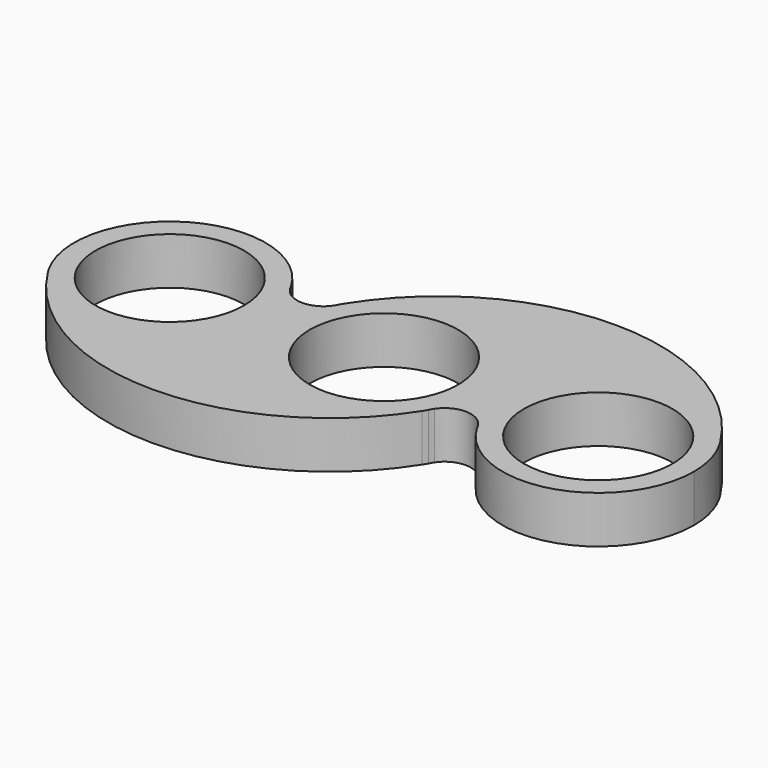
from build123d import *

# Parameters (mm, degrees)
F0_R     = 11.0109
F1_DEPTH = 7


with BuildPart() as f1:
    # F0 (on Top) → F1 (new body)
    with BuildSketch(Plane.XY):
        with BuildLine():
            Line((14.1859, 0), (11.0109, 0))
            ThreePointArc((11.0109, 0), (0, -11.0109), (-11.0109, 0))
            Line((-11.0109, 0), (-14.1859, 0))
            ThreePointArc((-14.1859, 0), (-4.0564627793, -13.5935598182), (11.8660062633, -7.7741658182))
            ThreePointArc((11.8660062633, -7.7741658182), (12.0777532722, -7.4348353952), (12.2853497755, -7.09295))
            ThreePointArc((12.2853497755, -7.09295), (12.4445825488, -6.7642227487), (12.6338376613, -6.4518140673))
            ThreePointArc((12.6338376613, -6.4518140673), (13.7924275689, -3.3179361907), (14.1859, 0))
        make_face()
        with BuildLine():
            ThreePointArc((-11.0109, 0), (0, 11.0109), (11.0109, 0))
            Line((11.0109, 0), (14.1859, 0))
            ThreePointArc((14.1859, 0), (4.0422659472, 13.5977882327), (-11.882216203, 7.7493675171))
            ThreePointArc((-11.882216203, 7.7493675171), (-12.0857093478, 7.4223418162), (-12.2853497755, 7.09295))
            ThreePointArc((-12.2853497755, 7.09295), (-12.4445825488, 6.7642227487), (-12.6338376613, 6.4518140673))
            ThreePointArc((-12.6338376613, 6.4518140673), (-13.7924275689, 3.3179361907), (-14.1859, 0))
            Line((-14.1859, 0), (-11.0109, 0))
        make_face()
        with BuildLine():
            Line((17.5641, 0), (14.1859, 0))
            ThreePointArc((14.1859, 0), (13.7924275689, -3.3179361907), (12.6338376613, -6.4518140673))
            ThreePointArc((12.6338376613, -6.4518140673), (15.875, -4.7244), (19.1161623387, -6.4518140673))
            ThreePointArc((19.1161623387, -6.4518140673), (17.9575724311, -3.3179361907), (17.5641, 0))
        make_face()
        with BuildLine():
            ThreePointArc((-11.882216203, 7.7493675171), (4.0422659472, 13.5977882327), (14.1859, 0))
            Line((14.1859, 0), (17.5641, 0))
            ThreePointArc((17.5641, 0), (27.7077340528, 13.5977882327), (43.632216203, 7.7493675171))
            ThreePointArc((43.632216203, 7.7493675171), (15.875, 23.0632), (-11.882216203, 7.7493675171))
        make_face()
        with BuildLine():
            Line((-17.5641, 0), (-14.1859, 0))
            ThreePointArc((-14.1859, 0), (-13.7924275689, 3.3179361907), (-12.6338376613, 6.4518140673))
            ThreePointArc((-12.6338376613, 6.4518140673), (-15.875, 4.7244), (-19.1161623387, 6.4518140673))
            ThreePointArc((-19.1161623387, 6.4518140673), (-17.9575724311, 3.3179361907), (-17.5641, 0))
        make_face()
        with BuildLine():
            ThreePointArc((11.8660062633, -7.7741658182), (-4.0564627793, -13.5935598182), (-14.1859, 0))
            Line((-14.1859, 0), (-17.5641, 0))
            ThreePointArc((-17.5641, 0), (-27.6935372207, -13.5935598182), (-43.6160062633, -7.7741658182))
            ThreePointArc((-43.6160062633, -7.7741658182), (-15.875, -23.0520875), (11.8660062633, -7.7741658182))
        make_face()
        with BuildLine():
            ThreePointArc((43.632216203, 7.7493675171), (27.7077340528, 13.5977882327), (17.5641, 0))
            ThreePointArc((17.5641, 0), (17.9575724311, -3.3179361907), (19.1161623387, -6.4518140673))
            ThreePointArc((19.1161623387, -6.4518140673), (19.3054174512, -6.7642227487), (19.4646502245, -7.09295))
            ThreePointArc((19.4646502245, -7.09295), (35.4215810919, -13.7025271792), (45.9359, 0))
            ThreePointArc((45.9359, 0), (45.4525271792, 3.6715810919), (44.0353497755, 7.09295))
            ThreePointArc((44.0353497755, 7.09295), (43.8357093478, 7.4223418162), (43.632216203, 7.7493675171))
        make_face()
        with BuildLine():
            ThreePointArc((42.7609, 0), (31.75, -11.0109), (20.7391, 0))
            ThreePointArc((20.7391, 0), (31.75, 11.0109), (42.7609, 0))
        make_face(mode=Mode.SUBTRACT)
        with BuildLine():
            ThreePointArc((-43.6160062633, -7.7741658182), (-27.6935372207, -13.5935598182), (-17.5641, 0))
            ThreePointArc((-17.5641, 0), (-17.9575724311, 3.3179361907), (-19.1161623387, 6.4518140673))
            ThreePointArc((-19.1161623387, 6.4518140673), (-19.3054174512, 6.7642227487), (-19.4646502245, 7.09295))
            ThreePointArc((-19.4646502245, 7.09295), (-38.84295, 12.2853497755), (-44.0353497755, -7.09295))
            ThreePointArc((-44.0353497755, -7.09295), (-43.8277532722, -7.4348353952), (-43.6160062633, -7.7741658182))
        make_face()
        with Locations((-31.75, 0)):
            Circle(F0_R, mode=Mode.SUBTRACT)
    extrude(amount=F1_DEPTH)


solid = f1.part
